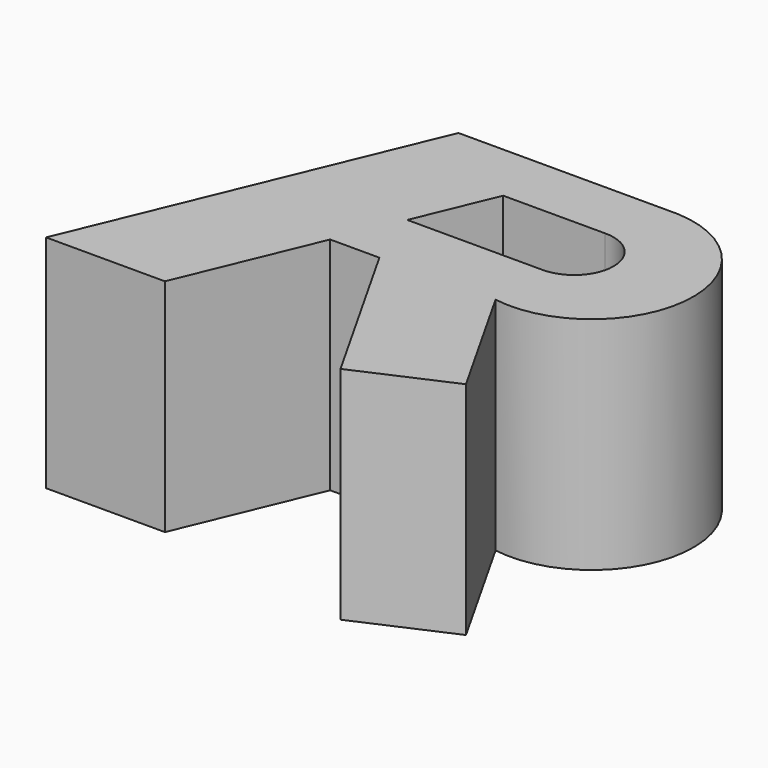
from build123d import *

# Parameters (mm, degrees)
F1_DEPTH = 12.7


# Not quite as in the source:
# - a feature names something its author has since deleted; it is built from what else it names


with BuildPart() as f1:
    # F0 (on Top) → F1 (new body)
    with BuildSketch(Plane.XY):
        with BuildLine():
            Line((63.0196762211, 10.9010377465), (50.3931596336, 10.9010377465))
            Line((50.3931596336, 10.9010377465), (42.2776843256, -8.6024441122))
            Line((42.2776843256, -8.6024441122), (49.1147374354, -8.6024441122))
            Line((49.1147374354, -8.6024441122), (52.3656376201, -0.7897319333))
            Line((52.3656376201, -0.7897319333), (55.199665187, -0.7897319333))
            Line((55.199665187, -0.7897319333), (60.5922424733, -10.3281843676))
            Line((60.5922424733, -10.3281843676), (65.9258010509, -7.9737302361))
            Line((65.9258010509, -7.9737302361), (61.8239495523, -0.7183283504))
            ThreePointArc((61.8239495523, -0.7183283504), (68.5532030557, 4.4603851012), (63.0196762211, 10.9010377465))
        make_face()
        with BuildLine():
            Line((53.8841895381, 2.8597215688), (55.7706488767, 7.3933470303))
            Line((55.7706488767, 7.3933470303), (61.637538461, 7.3933470303))
            ThreePointArc((61.637538461, 7.3933470303), (63.9369023486, 5.1428976256), (61.6700313985, 2.8597215688))
            Line((61.6700313985, 2.8597215688), (53.8841895381, 2.8597215688))
        make_face(mode=Mode.SUBTRACT)
    extrude(amount=F1_DEPTH)


solid = f1.part
